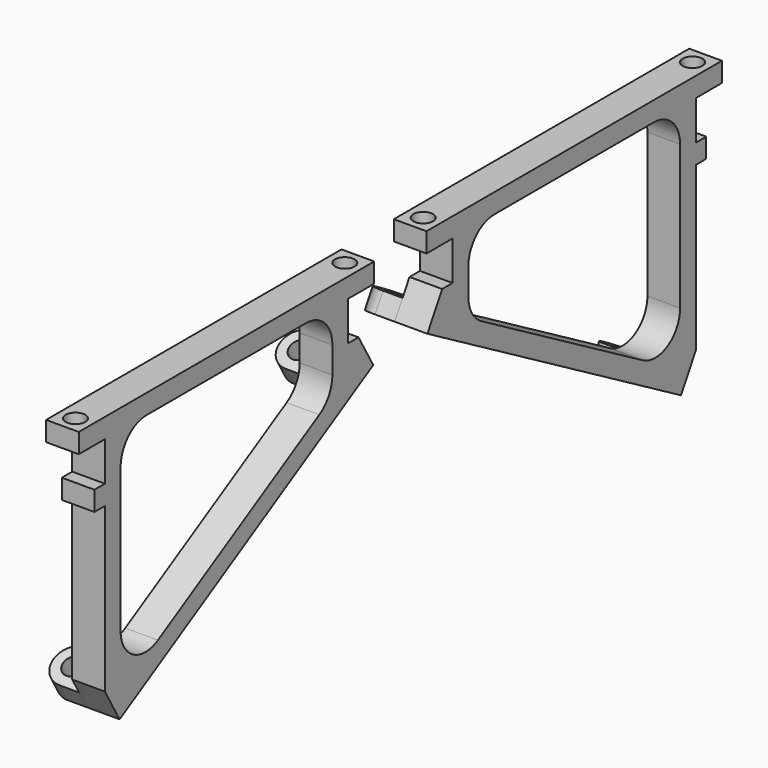
from build123d import *

# Parameters (mm, degrees)
F1_DEPTH = 5
F3_DEPTH = 6
F4_R     = 1.5
F5_DEPTH = 3
F6_R     = 1.5
F7_DEPTH = 25
F8_R     = 2.99999


# Not quite as in the source:
# - a fillet or chamfer is up to 0.001 mm smaller than in the source, because OpenCascade refuses the exact size


with BuildPart() as f1:
    # F0 (on Right) → F1 (new body)
    with BuildSketch(Plane.YZ):
        Polygon((15, 0), (0, 0), (0, -3), (5, -3), (5, -9), (3, -9), (0.1797888042, -13.8847490792), (48.6772114161, -41.8847490792), (51.4974226119, -37), (51.4974226119, -12), (53.4974226119, -12), (53.4974226119, -9), (51.4974226119, -9), (51.4974226119, -3), (56.4974226119, -3), (56.4974226119, 0), (48.4974226119, 0), align=None)
        with BuildLine():
            ThreePointArc((48.4974226119, -30.0741666773), (46.1179659481, -34.1955065134), (41.3590526205, -34.1955065134))
            Line((41.3590526205, -34.1955065134), (10.5, -16.3790241761))
            ThreePointArc((10.5, -16.3790241761), (8.6698729811, -14.5488971571), (8, -12.0488971571))
            Line((8, -12.0488971571), (8, -8))
            ThreePointArc((8, -8), (9.4644660941, -4.4644660941), (13, -3))
            Line((13, -3), (20, -3))
            Line((20, -3), (43.4974226119, -3))
            ThreePointArc((43.4974226119, -3), (47.0329565179, -4.4644660941), (48.4974226119, -8))
            Line((48.4974226119, -8), (48.4974226119, -12))
            Line((48.4974226119, -12), (48.4974226119, -30.0741666773))
        make_face(mode=Mode.SUBTRACT)
    extrude(amount=F1_DEPTH)

    # F2 (on face) → F3 (join)
    with BuildSketch(Plane(origin=(0, 0, 0), x_dir=(0, -1, 0), z_dir=(-1, 0, 0))):
        Polygon((-6.8759412269, -14.2866728679), (-5.3759412269, -16.8847490792), (-0.1797888042, -13.8847490792), (-1.6797888042, -11.2866728679), align=None)
        Polygon((-50.1772114161, -39.2866728679), (-48.6772114161, -41.8847490792), (-43.4810589934, -38.8847490792), (-44.981060144, -36.2866721082), align=None)
    extrude(amount=F3_DEPTH)

    # F4 (on face) → F5 (cut, through all)
    with BuildSketch(Plane.XY):
        with Locations((2.5, 2.5)):
            Circle(F4_R)
        with Locations((2.5, 53.9974226119)):
            Circle(F4_R)
    extrude(amount=-F5_DEPTH, mode=Mode.SUBTRACT)

    # F6 (on face) → F7 (cut)
    with BuildSketch(Plane(origin=(0, -5.9673255128, -10.3357109735), x_dir=(1, 0, 0), z_dir=(0, -0.5, -0.8660254038))):
        with Locations((-3, -10.0980762114)):
            Circle(F6_R)
        with Locations((-3, -60.0980762114)):
            Circle(F6_R)
    extrude(amount=-F7_DEPTH, mode=Mode.SUBTRACT)

    # F8 (radius 3 in the source; OpenCascade refuses exactly that, so slightly less here)
    f8_edges = [f1.edges().sort_by_distance(p)[0] for p in [
        (-6, 0.929789, -12.585711),
        (-6, 6.125941, -15.585711),
        (-6, 44.23106, -37.585711),
        (-6, 49.427211, -40.585711),
    ]]
    fillet(f8_edges, radius=F8_R)


with BuildPart() as f10_1:
    # F10: instance of F1
    add(f1.part.mirror(Plane.XZ.offset(5)))


solid = Compound([f1.part, f10_1.part])
